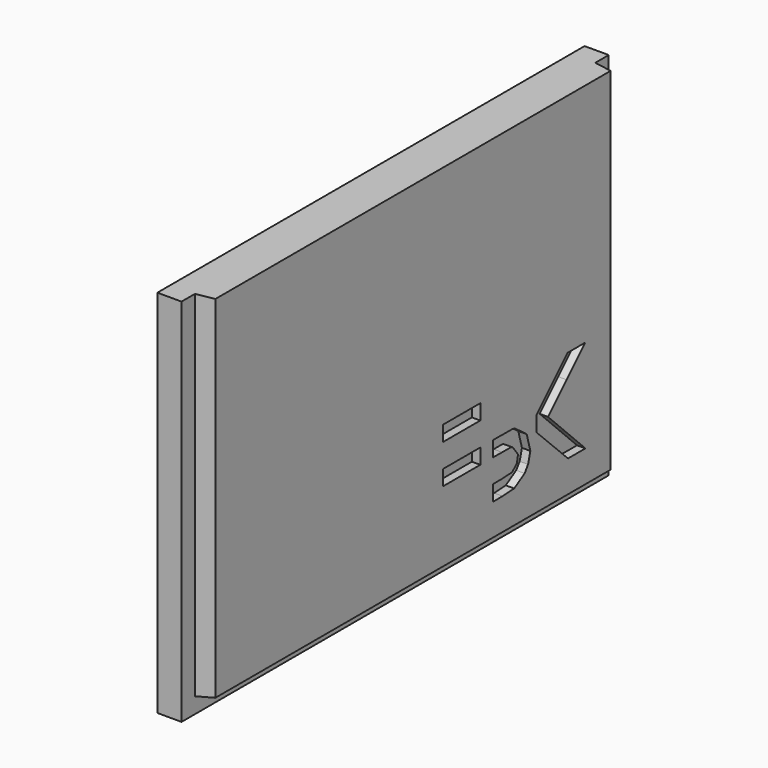
from build123d import *

# Parameters (mm, degrees)
F0_W         = 1.7
F0_H         = 47.6
F1_DEPTH     = 35.2
F2_DEPTH     = 1.5
F3_T4_DEPTH  = 42.5422275002
F3_T9_DEPTH  = 56.4422275002
F3_T14_DEPTH = 42.5422275002
F5_DEPTH     = 0.8


# Not quite as in the source:
# - a fillet or chamfer that OpenCascade refuses, or shapes differently, is made with other operations: its cross-section is extruded or revolved along the edge and cut away or added
# - ends of sketch curves that miss each other by under 0.0002 mm in the source are joined


with BuildPart() as f1:
    # F0 (on Top) → F1 (new body)
    with BuildSketch(Plane.XY):
        Polygon((21.457163617, -2.1686828911), (21.457163617, -52.9686828911), (23.757163617, -52.9686828911), (23.757163617, -51.3686828911), (23.757163617, -3.7686828911), (23.757163617, -2.1686828911), align=None)
        with Locations((24.607163617, -27.5686828911)):
            Rectangle(F0_W, F0_H)
    extrude(amount=F1_DEPTH)

    # F0 (on Top) → F2 (cut)
    with BuildSketch(Plane.XY):
        with Locations((24.607163617, -27.5686828911)):
            Rectangle(F0_W, F0_H)
    extrude(amount=F2_DEPTH, mode=Mode.SUBTRACT)

    # F3: chamfer of 0.3 x 1.7013845459 on 3 edges, made by hand


with BuildPart() as f3_tool2:
    # F3_s3 → F3_t4 (new body)
    with BuildSketch(Plane.XY.offset(-2.9211137501)):
        Polygon((25.457163617, -51.0686828911), (23.7557790711, -51.3686828911), (25.457163617, -51.3686828911), align=None)
    extrude(amount=F3_T4_DEPTH)

    split(bisect_by=Plane.YZ.offset(23.757163617), keep=Keep.TOP)


with BuildPart() as f1_1:
    add(f1.part)

    # F3_t1: cut F3_tool2
    add(f3_tool2.part, mode=Mode.SUBTRACT)


with BuildPart() as f3_tool7:
    # F3_s8 → F3_t9 (new body)
    with BuildSketch(Plane.XZ.offset(55.7897966412)):
        Polygon((23.7557790711, 1.5), (25.457163617, 1.8), (25.457163617, 1.5), align=None)
    extrude(amount=-F3_T9_DEPTH)

    split(bisect_by=Plane.YZ.offset(23.757163617), keep=Keep.TOP)


with BuildPart() as f1_2:
    add(f1_1.part)

    # F3_t6: cut F3_tool7
    add(f3_tool7.part, mode=Mode.SUBTRACT)


with BuildPart() as f3_tool12:
    # F3_s13 → F3_t14 (new body)
    with BuildSketch(Plane.XY.offset(-2.9211137501)):
        Polygon((23.7557790711, -3.7686828911), (25.457163617, -4.0686828911), (25.457163617, -3.7686828911), align=None)
    extrude(amount=F3_T14_DEPTH)

    split(bisect_by=Plane.YZ.offset(23.757163617), keep=Keep.TOP)


with BuildPart() as f1_3:
    add(f1_2.part)

    # F3_t11: cut F3_tool12
    add(f3_tool12.part, mode=Mode.SUBTRACT)

    # F4 (on face) → F5 (cut)
    with BuildSketch(Plane.YZ.offset(25.457163617)):
        Polygon((-24.0221414911, 13.6708992), (-24.0221414911, 12.9445354), (-24.0221414911, 12.2181716), (-21.7966950911, 12.2181716), (-19.5712486911, 12.2181716), (-19.5712486911, 12.9445354), (-19.5712486911, 13.6708992), (-21.7966950911, 13.6708992), align=None)
        Polygon((-24.0221414911, 9.9618134), (-24.0221414911, 9.2354496), (-24.0221414911, 8.5090858), (-21.7966950911, 8.5090858), (-19.5712486911, 8.5090858), (-19.5712486911, 9.2354496), (-19.5712486911, 9.9618134), (-21.7966950911, 9.9618134), align=None)
        Polygon((-18.0566974911, 6.280566), (-18.0566974911, 5.5376414), (-18.0566974911, 4.7947676), (-16.9207840911, 4.807493), (-15.5376016911, 4.8880872), (-14.2955670911, 5.6452866), (-13.8898274911, 6.2280134), (-13.6151518911, 7.2483822), (-14.0528446911, 8.8343074), (-15.3985112911, 9.8445416), (-15.6921352911, 9.9462178), (-16.8744290911, 9.9559968), (-18.0566974911, 9.9658012), (-18.0566974911, 9.2389548), (-18.0566974911, 8.512083), (-16.9818456911, 8.5028628), (-15.9070192911, 8.4936172), (-15.7007458911, 8.3920426), (-15.0843894911, 7.5677364), (-15.2217272911, 6.8451064), (-15.7842102911, 6.3483586), (-17.0050104911, 6.2828266), align=None)
        Polygon((-12.8639722911, 8.4833048), (-11.0016950911, 6.6416524), (-9.1394178911, 4.8), (-8.1040376911, 4.8), (-7.0686828911, 4.8), (-9.2939768911, 7.0254464), (-11.5192454911, 9.2508928), (-9.3094200911, 11.460896), (-7.0995692911, 13.6708992), (-8.1350510911, 13.6708992), (-9.1705328911, 13.6708992), (-11.0172398911, 11.823989), (-12.8639722911, 9.9770788), (-12.8639722911, 9.2301918), align=None)
    extrude(amount=-F5_DEPTH, mode=Mode.SUBTRACT)


solid = f1_3.part
